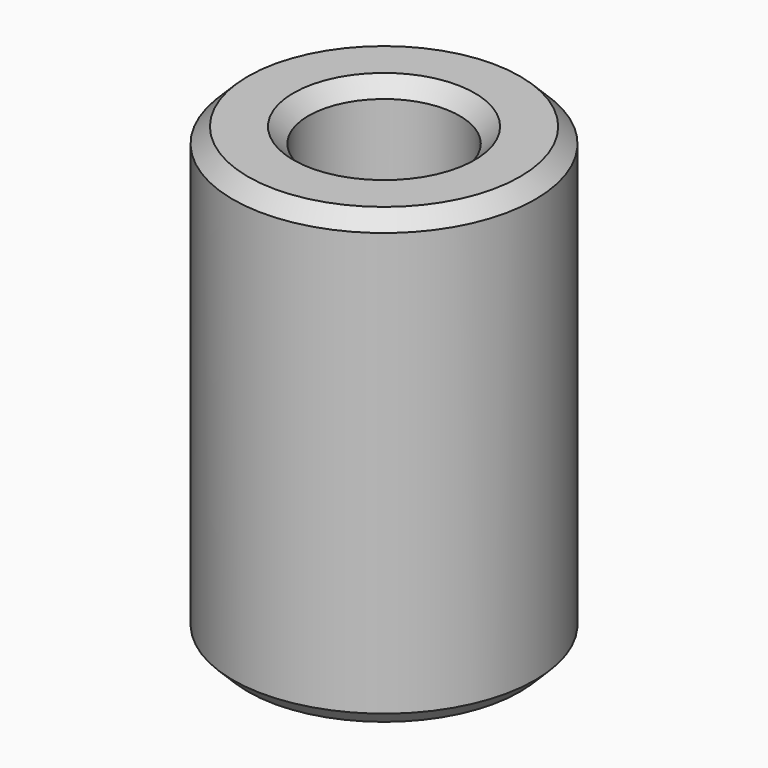
from build123d import *

# Parameters (mm, degrees)
F0_R     = 10
F1_DEPTH = 30
F3_D     = 10
F4_SIZE  = 1


with BuildPart() as f1:
    # F0 (on Top) → F1 (new body)
    with BuildSketch(Plane.XY):
        Circle(F0_R)
    extrude(amount=F1_DEPTH)

    # F3 (through all)
    with Locations(Plane(origin=(0, 0, 0), x_dir=(1, 0, 0), z_dir=(0, 0, -1))):
        with Locations((0, 0)):
            Hole(F3_D / 2)

    # F4
    f4_edges = [f1.edges().sort_by_distance(p)[0] for p in [
        (10, 0, 15),
        (-10, 0, 0),
        (-10, 0, 30),
        (-5, 0, 0),
        (-5, 0, 30),
    ]]
    chamfer(f4_edges, length=F4_SIZE)


solid = f1.part
